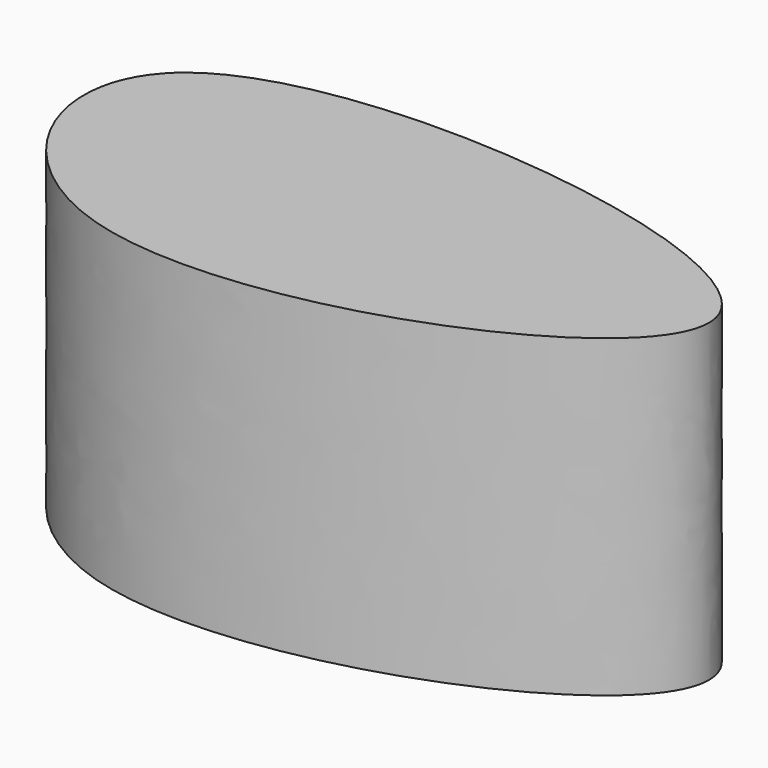
from build123d import *

# Parameters (mm, degrees)
F1_DEPTH = 25.4


with BuildPart() as f1:
    # F0 (on Top) → F1 (new body)
    with BuildSketch(Plane.XY):
        with BuildLine():
            add(Edge.make_bspline(
                [(-27.3207575083, 55.0033822656), (-17.4990871634, 62.9767087539), (49.7782982933, 53.9519843925), (-22.7022690183, 23.2303922467), (-33.9235899615, 49.6431393487), (-27.3207575083, 55.0033822656)],
                knots=[0, 0, 0, 0, 0.3841528315, 0.7417448668, 1, 1, 1, 1], degree=3))
        make_face()
    extrude(amount=F1_DEPTH)


solid = f1.part
